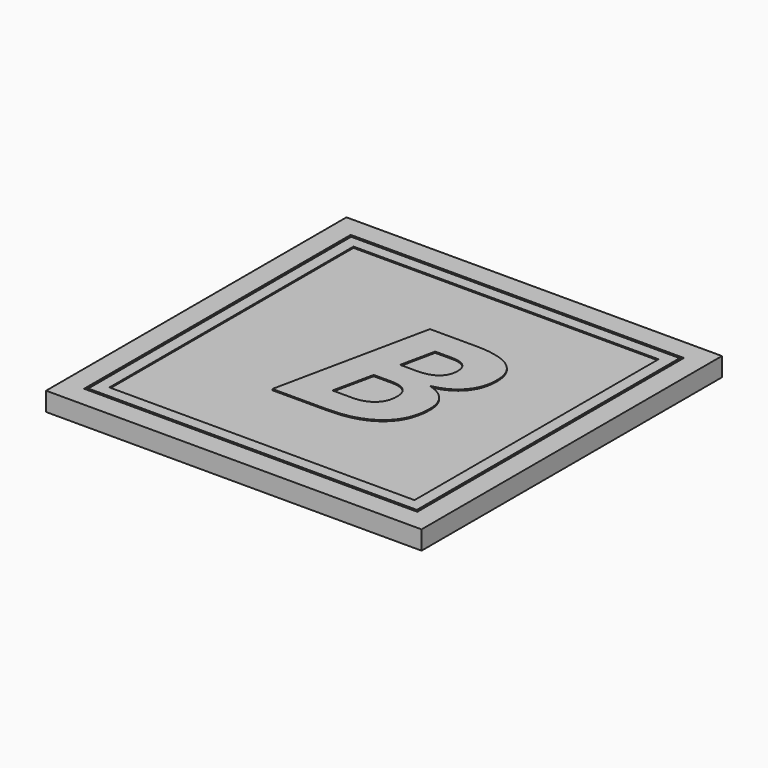
from build123d import *

# Parameters (mm, degrees)
F0_W         = 101.6
F0_H         = 101.6
F1_DEPTH     = 5.08
F2_W         = 90.17
F2_H         = 90.17
F2_W_2       = 88.9
F2_H_2       = 88.9
F3_DEPTH     = 0.254
F4_W         = 82.55
F4_H         = 82.55
F5_DEPTH     = 0.3175
F6_TEXT_SIZE = 59.081800282
F7_DEPTH     = 0.3175


# Not quite as in the source:
# - Text() gives the source's letters only with a copy of the font that has no kerning and outlines rounded to 1/6400 em; it was checked with that copy


with BuildPart() as f1:
    # F0 (on Top) → F1 (new body)
    with BuildSketch(Plane.XY):
        with Locations((-22.9751824458, -0.2391925082)):
            Rectangle(F0_W, F0_H)
    extrude(amount=F1_DEPTH)

    # F2 (on face) → F3 (cut)
    with BuildSketch(Plane.XY.offset(5.08)):
        with Locations((-22.9751824458, -0.2391925082)):
            Rectangle(F2_W, F2_H)
        with Locations((-22.9751824458, -0.2391925082)):
            Rectangle(F2_W_2, F2_H_2, mode=Mode.SUBTRACT)
    extrude(amount=-F3_DEPTH, mode=Mode.SUBTRACT)

    # F4 (on face) → F5 (cut)
    with BuildSketch(Plane.XY.offset(5.08)):
        with Locations((-22.9751824458, -0.2391925082)):
            Rectangle(F4_W, F4_H)
    extrude(amount=-F5_DEPTH, mode=Mode.SUBTRACT)

    # F6 (on face) → F7 (join, through all)
    with BuildSketch(Plane.XY.offset(4.7625)):
        with Locations((-38.4747311473, -20.5469215289)):
            Text('B', F6_TEXT_SIZE, font='Open Sans', font_style=FontStyle.BOLDITALIC, text_align=(TextAlign.LEFT, TextAlign.BOTTOM))
    extrude(amount=F7_DEPTH)


solid = f1.part
